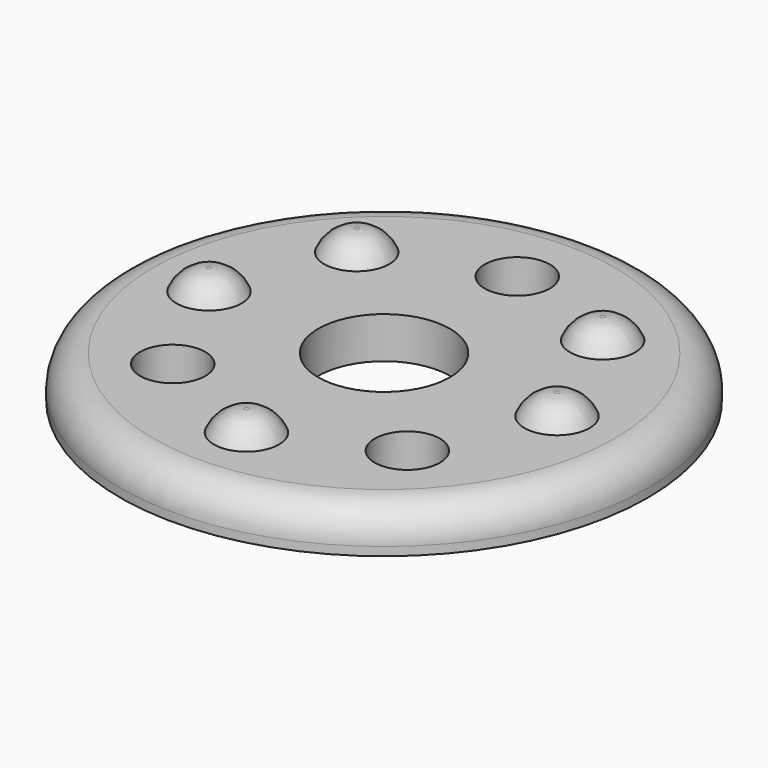
from build123d import *

# Parameters (mm, degrees)
F0_R     = 44.5
F0_R_2   = 5.5
F0_R_3   = 11.1
F1_DEPTH = 7
F2_R     = 5.5526911935
F3_R     = 5.5
F4_DEPTH = 3.5


# Not quite as in the source:
# - a fillet or chamfer that OpenCascade refuses, or shapes differently, is made with other operations: its cross-section is extruded or revolved along the edge and cut away or added


with BuildPart() as f1:
    # F0 (on Top) → F1 (new body)
    with BuildSketch(Plane.XY):
        with Locations((1.3388e-06, 0.0960128228)):
            Circle(F0_R)
        with Locations((-19.7783853119, -19.7235588551)):
            Circle(F0_R_2, mode=Mode.SUBTRACT)
        with Locations((19.7783879895, -19.7235588551)):
            Circle(F0_R_2, mode=Mode.SUBTRACT)
        with Locations((1.3388e-06, 0.0960128228)):
            Circle(F0_R_3, mode=Mode.SUBTRACT)
        with Locations((0.0567746402, 28.095976607)):
            Circle(F0_R_2, mode=Mode.SUBTRACT)
    extrude(amount=F1_DEPTH)

    # F2
    f2_edges = [f1.edges().sort_by_distance(p)[0] for p in [
        (-44.499999, 0.096013, 7),
    ]]
    fillet(f2_edges, radius=F2_R)

    # F3 (on face) → F4 (join)
    with BuildSketch(Plane.XY.offset(7)):
        with Locations((20.2050062432, 20.8988438036)):
            Circle(F3_R)
        with Locations((28.9993370366, 0.292301098)):
            Circle(F3_R)
        with Locations((1.3388e-06, -28.9039871772)):
            Circle(F3_R)
        with Locations((-28.9925298787, -0.5621160422)):
            Circle(F3_R)
        with Locations((-20.7871988103, 20.3170985988)):
            Circle(F3_R)
    extrude(amount=F4_DEPTH)

    # F5: fillet of radius 5.5 on 5 edges, made by hand

    # F5_s1 → F5_t2 (revolve, cut)
    with BuildSketch(Plane.XZ.offset(0.5621160422)):
        with BuildLine():
            ThreePointArc((-23.4925298787, 7), (-25.5135868502, 9.5414755311), (-28.6160052617, 10.5))
            Line((-28.6160052617, 10.5), (-23.4925298787, 10.5))
            Line((-23.4925298787, 10.5), (-23.4925298787, 7))
        make_face()
    revolve(axis=Axis((-28.9925298787, -0.5621160422, 10.5), (0, 0, 1)), mode=Mode.SUBTRACT)

    # F5_s3 → F5_t4 (revolve, cut)
    with BuildSketch(Plane.XZ.offset(-20.3170985988)):
        with BuildLine():
            ThreePointArc((-15.2871988103, 7), (-17.3082557818, 9.5414755311), (-20.4106741933, 10.5))
            Line((-20.4106741933, 10.5), (-15.2871988103, 10.5))
            Line((-15.2871988103, 10.5), (-15.2871988103, 7))
        make_face()
    revolve(axis=Axis((-20.7871988103, 20.3170985988, 10.5), (0, 0, 1)), mode=Mode.SUBTRACT)

    # F5_s5 → F5_t6 (revolve, cut)
    with BuildSketch(Plane.XZ.offset(-20.8988438036)):
        with BuildLine():
            ThreePointArc((25.7050062432, 7), (23.6839492717, 9.5414755311), (20.5815308602, 10.5))
            Line((20.5815308602, 10.5), (25.7050062432, 10.5))
            Line((25.7050062432, 10.5), (25.7050062432, 7))
        make_face()
    revolve(axis=Axis((20.2050062432, 20.8988438036, 10.5), (0, 0, 1)), mode=Mode.SUBTRACT)

    # F5_s7 → F5_t8 (revolve, cut)
    with BuildSketch(Plane.XZ.offset(-0.292301098)):
        with BuildLine():
            ThreePointArc((34.4993370366, 7), (32.4782800651, 9.5414755311), (29.3758616536, 10.5))
            Line((29.3758616536, 10.5), (34.4993370366, 10.5))
            Line((34.4993370366, 10.5), (34.4993370366, 7))
        make_face()
    revolve(axis=Axis((28.9993370366, 0.292301098, 10.5), (0, 0, 1)), mode=Mode.SUBTRACT)

    # F5_s9 → F5_t10 (revolve, cut)
    with BuildSketch(Plane.XZ.offset(28.9039871772)):
        with BuildLine():
            ThreePointArc((5.5000013388, 7), (3.4789443673, 9.5414755311), (0.3765259558, 10.5))
            Line((0.3765259558, 10.5), (5.5000013388, 10.5))
            Line((5.5000013388, 10.5), (5.5000013388, 7))
        make_face()
    revolve(axis=Axis((1.3388e-06, -28.9039871772, 10.5), (0, 0, 1)), mode=Mode.SUBTRACT)


solid = f1.part
